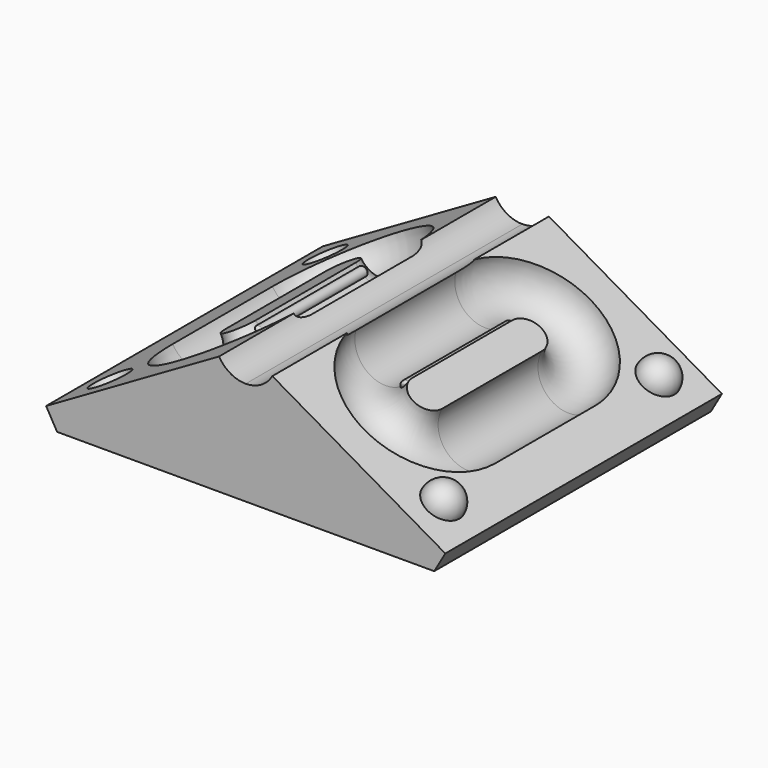
from build123d import *

# Parameters (mm, degrees)
F1_DEPTH  = 9
F3_R      = 1.6
F5_R      = 0.2664132943
F6_DEPTH  = 3.5
F7_R      = 0.15
F9_R      = 1
F10_DEPTH = 1
F11_R     = 0.99999
F12_R     = 1
F13_DEPTH = 1
F14_R     = 0.99999


# Not quite as in the source:
# - a fillet or chamfer is up to 0.001 mm smaller than in the source, because OpenCascade refuses the exact size


with BuildPart() as f1:
    # F0 (on Front) → F1 (new body, symmetric)
    with BuildSketch(Plane.XZ):
        with BuildLine():
            Line((0, 5.4), (0, 0))
            Line((0, 0), (9.8149545762, 0))
            Line((9.8149545762, 0), (10.3923048454, 1))
            Line((10.3923048454, 1), (1.3856406461, 6.2))
            ThreePointArc((1.3856406461, 6.2), (0.8, 5.6143593539), (0, 5.4))
        make_face()
    extrude(amount=F1_DEPTH, both=True)

    # F4: sweep along a path in F2
    with BuildLine(Plane(origin=(3.0310889132, 0, 5.25), x_dir=(0.8660254038, 0, -0.5), z_dir=(0.5, 0, 0.8660254038))) as f4_path:
        Line((-0.4, 0), (-0.4, -3.25))
        ThreePointArc((-0.4, -3.25), (2.1, -5.75), (4.6, -3.25))
        Line((4.6, -3.25), (4.6, 0))
        Line((4.6, 0), (4.6, 3.25))
        ThreePointArc((4.6, 3.25), (2.1, 5.75), (-0.4, 3.25))
        Line((-0.4, 3.25), (-0.4, 0))
    # F3 (on Front) → F4 (sweep, cut)
    with BuildSketch(Plane.XZ):
        with Locations((2.6846787517, 5.45)):
            Circle(F3_R)
    sweep(path=f4_path.line, mode=Mode.SUBTRACT)

    # F5 (on Front) → F6 (join, symmetric)
    with BuildSketch(Plane.XZ):
        with Locations((3.8403375997, 4.2442123709)):
            Circle(F5_R)
    extrude(amount=F6_DEPTH, both=True)

    # F7
    f7_edges = [f1.edges().sort_by_distance(p)[0] for p in [
        (3.658788, -3.5, 4.439188),
        (3.658788, 3.5, 4.439188),
    ]]
    fillet(f7_edges, radius=F7_R)

    # F8: F1 across plane


with BuildPart() as f1_1:
    add(f1.part)
    add(f1.part.mirror(Plane.YZ))

    # F9 (on face) → F10 (join)
    with BuildSketch(Plane(origin=(3.0310889132, 0, 5.25), x_dir=(0.8660254038, 0, -0.5), z_dir=(0.5, 0, 0.8660254038))):
        with Locations((6.5, 7)):
            Circle(F9_R)
        with Locations((6.5, -7)):
            Circle(F9_R)
    extrude(amount=F10_DEPTH)

    # F11 (radius 1 in the source; OpenCascade refuses exactly that, so slightly less here)
    f11_edges = [f1_1.edges().sort_by_distance(p)[0] for p in [
        (8.294229, 7, 3.366025),
        (8.294229, -7, 3.366025),
    ]]
    fillet(f11_edges, radius=F11_R)

    # F12 (on face) → F13 (cut)
    with BuildSketch(Plane(origin=(-3.0310889132, 0, 5.25), x_dir=(0.8660254038, 0, 0.5), z_dir=(-0.5, 0, 0.8660254038))):
        with Locations((-6.5, 7)):
            Circle(F12_R)
        with Locations((-6.5, -7)):
            Circle(F12_R)
    extrude(amount=-F13_DEPTH, mode=Mode.SUBTRACT)

    # F14 (radius 1 in the source; OpenCascade refuses exactly that, so slightly less here)
    f14_edges = [f1_1.edges().sort_by_distance(p)[0] for p in [
        (-9.026279, 7, 0.633975),
        (-9.026279, -7, 0.633975),
    ]]
    fillet(f14_edges, radius=F14_R)


solid = f1_1.part
